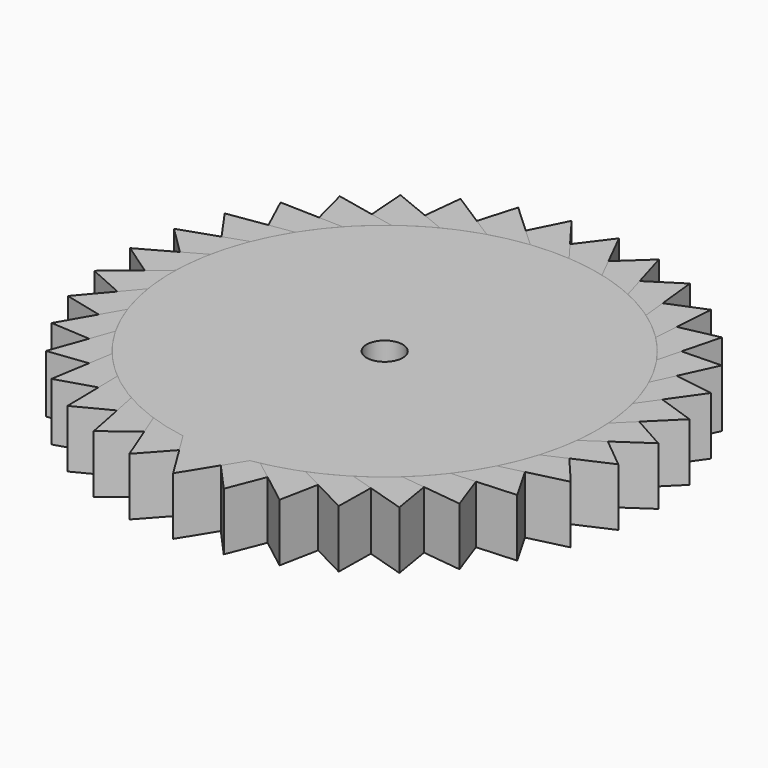
from build123d import *

# Parameters (mm, degrees)
F1_DEPTH = 10.16
F2_COUNT = 35
F4_D     = 6.35
F4_2_D   = 6.35
F4_3_D   = 6.35
F4_4_D   = 6.35
F4_5_D   = 6.35
F4_6_D   = 6.35
F4_7_D   = 6.35
F4_8_D   = 6.35
F4_9_D   = 6.35
F4_10_D  = 6.35
F4_11_D  = 6.35
F4_12_D  = 6.35
F4_13_D  = 6.35
F4_14_D  = 6.35
F4_15_D  = 6.35
F4_16_D  = 6.35
F4_17_D  = 6.35
F4_18_D  = 6.35
F4_19_D  = 6.35
F4_20_D  = 6.35
F4_21_D  = 6.35
F4_22_D  = 6.35
F4_23_D  = 6.35
F4_24_D  = 6.35
F4_25_D  = 6.35
F4_26_D  = 6.35
F4_27_D  = 6.35
F4_28_D  = 6.35
F4_29_D  = 6.35
F4_30_D  = 6.35
F4_31_D  = 6.35
F4_32_D  = 6.35
F4_33_D  = 6.35
F4_34_D  = 6.35
F4_35_D  = 6.35


with BuildPart() as f1:
    # F0 (on Top) → F1 (new body)
    with BuildSketch(Plane.XY):
        with BuildLine():
            ThreePointArc((5.8892677334, -36.9507230084), (28.4640011907, -24.286622686), (37.4171004392, 0))
            ThreePointArc((37.4171004392, 0), (-24.286622686, 28.4640011907), (-5.8892677334, -36.9507230084))
            ThreePointArc((-5.8892677334, -36.9507230084), (-2.9538526683, -37.300323855), (0, -37.4171004392))
            ThreePointArc((0, -37.4171004392), (2.9538526683, -37.300323855), (5.8892677334, -36.9507230084))
        make_face()
        with BuildLine():
            Line((0, -46.4704111218), (5.8892677334, -36.9507230084))
            ThreePointArc((5.8892677334, -36.9507230084), (2.9538526683, -37.300323855), (0, -37.4171004392))
            Line((0, -37.4171004392), (0, -46.4704111218))
        make_face()
        with BuildLine():
            ThreePointArc((0, -37.4171004392), (-2.9538526683, -37.300323855), (-5.8892677334, -36.9507230084))
            Line((-5.8892677334, -36.9507230084), (0, -46.4704111218))
            Line((0, -46.4704111218), (0, -37.4171004392))
        make_face()
    extrude(amount=F1_DEPTH)


with BuildPart() as f2_1:
    # F2: instance of F1
    add(f1.part.rotate(Axis((0, 0, 0), (0, 0, 1)), 1 * 360 / F2_COUNT))

    # F4#2 (through all)
    with Locations(Plane.XY.offset(10.16)):
        with Locations((0, 0)):
            Hole(F4_2_D / 2)


with BuildPart() as f2_2:
    # F2: instance of F1
    add(f1.part.rotate(Axis((0, 0, 0), (0, 0, 1)), 2 * 360 / F2_COUNT))

    # F4#3 (through all)
    with Locations(Plane.XY.offset(10.16)):
        with Locations((0, 0)):
            Hole(F4_3_D / 2)


with BuildPart() as f2_3:
    # F2: instance of F1
    add(f1.part.rotate(Axis((0, 0, 0), (0, 0, 1)), 3 * 360 / F2_COUNT))

    # F4#4 (through all)
    with Locations(Plane.XY.offset(10.16)):
        with Locations((0, 0)):
            Hole(F4_4_D / 2)


with BuildPart() as f2_4:
    # F2: instance of F1
    add(f1.part.rotate(Axis((0, 0, 0), (0, 0, 1)), 4 * 360 / F2_COUNT))

    # F4#5 (through all)
    with Locations(Plane.XY.offset(10.16)):
        with Locations((0, 0)):
            Hole(F4_5_D / 2)


with BuildPart() as f2_5:
    # F2: instance of F1
    add(f1.part.rotate(Axis((0, 0, 0), (0, 0, 1)), 5 * 360 / F2_COUNT))

    # F4#6 (through all)
    with Locations(Plane.XY.offset(10.16)):
        with Locations((0, 0)):
            Hole(F4_6_D / 2)


with BuildPart() as f2_6:
    # F2: instance of F1
    add(f1.part.rotate(Axis((0, 0, 0), (0, 0, 1)), 6 * 360 / F2_COUNT))

    # F4#7 (through all)
    with Locations(Plane.XY.offset(10.16)):
        with Locations((0, 0)):
            Hole(F4_7_D / 2)


with BuildPart() as f2_7:
    # F2: instance of F1
    add(f1.part.rotate(Axis((0, 0, 0), (0, 0, 1)), 7 * 360 / F2_COUNT))

    # F4#8 (through all)
    with Locations(Plane.XY.offset(10.16)):
        with Locations((0, 0)):
            Hole(F4_8_D / 2)


with BuildPart() as f2_8:
    # F2: instance of F1
    add(f1.part.rotate(Axis((0, 0, 0), (0, 0, 1)), 8 * 360 / F2_COUNT))

    # F4#9 (through all)
    with Locations(Plane.XY.offset(10.16)):
        with Locations((0, 0)):
            Hole(F4_9_D / 2)


with BuildPart() as f2_9:
    # F2: instance of F1
    add(f1.part.rotate(Axis((0, 0, 0), (0, 0, 1)), 9 * 360 / F2_COUNT))

    # F4#10 (through all)
    with Locations(Plane.XY.offset(10.16)):
        with Locations((0, 0)):
            Hole(F4_10_D / 2)


with BuildPart() as f2_10:
    # F2: instance of F1
    add(f1.part.rotate(Axis((0, 0, 0), (0, 0, 1)), 10 * 360 / F2_COUNT))

    # F4#11 (through all)
    with Locations(Plane.XY.offset(10.16)):
        with Locations((0, 0)):
            Hole(F4_11_D / 2)


with BuildPart() as f2_11:
    # F2: instance of F1
    add(f1.part.rotate(Axis((0, 0, 0), (0, 0, 1)), 11 * 360 / F2_COUNT))

    # F4#12 (through all)
    with Locations(Plane.XY.offset(10.16)):
        with Locations((0, 0)):
            Hole(F4_12_D / 2)


with BuildPart() as f2_12:
    # F2: instance of F1
    add(f1.part.rotate(Axis((0, 0, 0), (0, 0, 1)), 12 * 360 / F2_COUNT))

    # F4#13 (through all)
    with Locations(Plane.XY.offset(10.16)):
        with Locations((0, 0)):
            Hole(F4_13_D / 2)


with BuildPart() as f2_13:
    # F2: instance of F1
    add(f1.part.rotate(Axis((0, 0, 0), (0, 0, 1)), 13 * 360 / F2_COUNT))

    # F4#14 (through all)
    with Locations(Plane.XY.offset(10.16)):
        with Locations((0, 0)):
            Hole(F4_14_D / 2)


with BuildPart() as f2_14:
    # F2: instance of F1
    add(f1.part.rotate(Axis((0, 0, 0), (0, 0, 1)), 14 * 360 / F2_COUNT))

    # F4#15 (through all)
    with Locations(Plane.XY.offset(10.16)):
        with Locations((0, 0)):
            Hole(F4_15_D / 2)


with BuildPart() as f2_15:
    # F2: instance of F1
    add(f1.part.rotate(Axis((0, 0, 0), (0, 0, 1)), 15 * 360 / F2_COUNT))

    # F4#16 (through all)
    with Locations(Plane.XY.offset(10.16)):
        with Locations((0, 0)):
            Hole(F4_16_D / 2)


with BuildPart() as f2_16:
    # F2: instance of F1
    add(f1.part.rotate(Axis((0, 0, 0), (0, 0, 1)), 16 * 360 / F2_COUNT))

    # F4#17 (through all)
    with Locations(Plane.XY.offset(10.16)):
        with Locations((0, 0)):
            Hole(F4_17_D / 2)


with BuildPart() as f2_17:
    # F2: instance of F1
    add(f1.part.rotate(Axis((0, 0, 0), (0, 0, 1)), 17 * 360 / F2_COUNT))

    # F4#18 (through all)
    with Locations(Plane.XY.offset(10.16)):
        with Locations((0, 0)):
            Hole(F4_18_D / 2)


with BuildPart() as f2_18:
    # F2: instance of F1
    add(f1.part.rotate(Axis((0, 0, 0), (0, 0, 1)), 18 * 360 / F2_COUNT))

    # F4#19 (through all)
    with Locations(Plane.XY.offset(10.16)):
        with Locations((0, 0)):
            Hole(F4_19_D / 2)


with BuildPart() as f2_19:
    # F2: instance of F1
    add(f1.part.rotate(Axis((0, 0, 0), (0, 0, 1)), 19 * 360 / F2_COUNT))

    # F4#20 (through all)
    with Locations(Plane.XY.offset(10.16)):
        with Locations((0, 0)):
            Hole(F4_20_D / 2)


with BuildPart() as f2_20:
    # F2: instance of F1
    add(f1.part.rotate(Axis((0, 0, 0), (0, 0, 1)), 20 * 360 / F2_COUNT))

    # F4#21 (through all)
    with Locations(Plane.XY.offset(10.16)):
        with Locations((0, 0)):
            Hole(F4_21_D / 2)


with BuildPart() as f2_21:
    # F2: instance of F1
    add(f1.part.rotate(Axis((0, 0, 0), (0, 0, 1)), 21 * 360 / F2_COUNT))

    # F4#22 (through all)
    with Locations(Plane.XY.offset(10.16)):
        with Locations((0, 0)):
            Hole(F4_22_D / 2)


with BuildPart() as f2_22:
    # F2: instance of F1
    add(f1.part.rotate(Axis((0, 0, 0), (0, 0, 1)), 22 * 360 / F2_COUNT))

    # F4#23 (through all)
    with Locations(Plane.XY.offset(10.16)):
        with Locations((0, 0)):
            Hole(F4_23_D / 2)


with BuildPart() as f2_23:
    # F2: instance of F1
    add(f1.part.rotate(Axis((0, 0, 0), (0, 0, 1)), 23 * 360 / F2_COUNT))

    # F4#24 (through all)
    with Locations(Plane.XY.offset(10.16)):
        with Locations((0, 0)):
            Hole(F4_24_D / 2)


with BuildPart() as f2_24:
    # F2: instance of F1
    add(f1.part.rotate(Axis((0, 0, 0), (0, 0, 1)), 24 * 360 / F2_COUNT))

    # F4#25 (through all)
    with Locations(Plane.XY.offset(10.16)):
        with Locations((0, 0)):
            Hole(F4_25_D / 2)


with BuildPart() as f2_25:
    # F2: instance of F1
    add(f1.part.rotate(Axis((0, 0, 0), (0, 0, 1)), 25 * 360 / F2_COUNT))

    # F4#26 (through all)
    with Locations(Plane.XY.offset(10.16)):
        with Locations((0, 0)):
            Hole(F4_26_D / 2)


with BuildPart() as f2_26:
    # F2: instance of F1
    add(f1.part.rotate(Axis((0, 0, 0), (0, 0, 1)), 26 * 360 / F2_COUNT))

    # F4#27 (through all)
    with Locations(Plane.XY.offset(10.16)):
        with Locations((0, 0)):
            Hole(F4_27_D / 2)


with BuildPart() as f2_27:
    # F2: instance of F1
    add(f1.part.rotate(Axis((0, 0, 0), (0, 0, 1)), 27 * 360 / F2_COUNT))

    # F4#28 (through all)
    with Locations(Plane.XY.offset(10.16)):
        with Locations((0, 0)):
            Hole(F4_28_D / 2)


with BuildPart() as f2_28:
    # F2: instance of F1
    add(f1.part.rotate(Axis((0, 0, 0), (0, 0, 1)), 28 * 360 / F2_COUNT))

    # F4#29 (through all)
    with Locations(Plane.XY.offset(10.16)):
        with Locations((0, 0)):
            Hole(F4_29_D / 2)


with BuildPart() as f2_29:
    # F2: instance of F1
    add(f1.part.rotate(Axis((0, 0, 0), (0, 0, 1)), 29 * 360 / F2_COUNT))

    # F4#30 (through all)
    with Locations(Plane.XY.offset(10.16)):
        with Locations((0, 0)):
            Hole(F4_30_D / 2)


with BuildPart() as f2_30:
    # F2: instance of F1
    add(f1.part.rotate(Axis((0, 0, 0), (0, 0, 1)), 30 * 360 / F2_COUNT))

    # F4#31 (through all)
    with Locations(Plane.XY.offset(10.16)):
        with Locations((0, 0)):
            Hole(F4_31_D / 2)


with BuildPart() as f2_31:
    # F2: instance of F1
    add(f1.part.rotate(Axis((0, 0, 0), (0, 0, 1)), 31 * 360 / F2_COUNT))

    # F4#32 (through all)
    with Locations(Plane.XY.offset(10.16)):
        with Locations((0, 0)):
            Hole(F4_32_D / 2)


with BuildPart() as f2_32:
    # F2: instance of F1
    add(f1.part.rotate(Axis((0, 0, 0), (0, 0, 1)), 32 * 360 / F2_COUNT))

    # F4#33 (through all)
    with Locations(Plane.XY.offset(10.16)):
        with Locations((0, 0)):
            Hole(F4_33_D / 2)


with BuildPart() as f2_33:
    # F2: instance of F1
    add(f1.part.rotate(Axis((0, 0, 0), (0, 0, 1)), 33 * 360 / F2_COUNT))

    # F4#34 (through all)
    with Locations(Plane.XY.offset(10.16)):
        with Locations((0, 0)):
            Hole(F4_34_D / 2)


with BuildPart() as f2_34:
    # F2: instance of F1
    add(f1.part.rotate(Axis((0, 0, 0), (0, 0, 1)), 34 * 360 / F2_COUNT))

    # F4#35 (through all)
    with Locations(Plane.XY.offset(10.16)):
        with Locations((0, 0)):
            Hole(F4_35_D / 2)


with BuildPart() as f1_1:
    add(f1.part)

    # F4 (through all)
    with Locations(Plane.XY.offset(10.16)):
        with Locations((0, 0)):
            Hole(F4_D / 2)


solid = Compound([f2_1.part, f2_2.part, f2_3.part, f2_4.part, f2_5.part, f2_6.part, f2_7.part, f2_8.part, f2_9.part, f2_10.part, f2_11.part, f2_12.part, f2_13.part, f2_14.part, f2_15.part, f2_16.part, f2_17.part, f2_18.part, f2_19.part, f2_20.part, f2_21.part, f2_22.part, f2_23.part, f2_24.part, f2_25.part, f2_26.part, f2_27.part, f2_28.part, f2_29.part, f2_30.part, f2_31.part, f2_32.part, f2_33.part, f2_34.part, f1_1.part])
